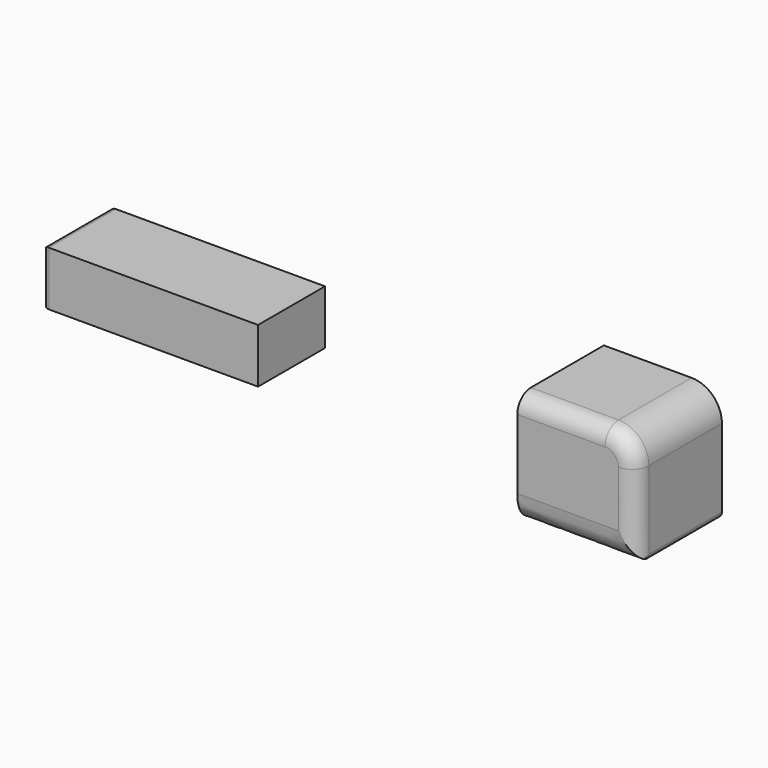
from build123d import *

# Parameters (mm, degrees)
F0_W        = 90.5269756913
F0_H        = 95.6492051482
F1_DEPTH    = 98.806
F2_R        = 25.4
F3_R        = 14.1038356314
F4_T1_DEPTH = 201.2121108887
F5_T1_DEPTH = 101.5149863872
F6_W        = 180.060595274
F6_H        = 70.0388215482
F7_DEPTH    = 45.466
F8_R        = 5.08


# Not quite as in the source:
# - a fillet or chamfer that OpenCascade refuses, or shapes differently, is made with other operations: its cross-section is extruded or revolved along the edge and cut away or added


with BuildPart() as f1:
    # F0 (on Right) → F1 (new body)
    with BuildSketch(Plane.YZ):
        with Locations((0.7718615234, 14.4452676177)):
            Rectangle(F0_W, F0_H)
    extrude(amount=F1_DEPTH)

    # F2
    f2_edges = [f1.edges().sort_by_distance(p)[0] for p in [
        (98.806, 0.771862, 62.26987),
    ]]
    fillet(f2_edges, radius=F2_R)

    # F3
    f3_edges = [f1.edges().sort_by_distance(p)[0] for p in [
        (36.703, -44.491626, 62.26987),
        (91.366512, -44.491626, 54.830382),
        (98.806, -44.491626, 1.745268),
    ]]
    fillet(f3_edges, radius=F3_R)

    # F4: fillet of radius 23.301989304 on 1 edges, made by hand

    # F4_s2 → F4_t1 (cut)
    with BuildSketch(Plane.YZ.offset(-58.2549732601)):
        with BuildLine():
            add(Edge.make_bspline(
                [(-44.4916263223, -10.0773456524), (-44.4916263223, -33.3793349564), (-21.1896370182, -33.3793349564)],
                knots=[0, 0, 0, 1, 1, 1], degree=2, weights=[1, 1, 1]))
            Line((-21.1896370182, -33.3793349564), (-44.4916263223, -33.3793349564))
            Line((-44.4916263223, -33.3793349564), (-44.4916263223, -10.0773456524))
        make_face()
    extrude(amount=F4_T1_DEPTH, mode=Mode.SUBTRACT)

    # F5: fillet of radius 5.08 on 1 edges, made by hand

    # F5_s2 → F5_t1 (cut)
    with BuildSketch(Plane.XZ.offset(-58.735349369)):
        with BuildLine():
            ThreePointArc((98.806, -28.2993349564), (97.3181024484, -31.8914374048), (93.726, -33.3793349564))
            Line((93.726, -33.3793349564), (98.806, -33.3793349564))
            Line((98.806, -33.3793349564), (98.806, -28.2993349564))
        make_face()
    extrude(amount=F5_T1_DEPTH, mode=Mode.SUBTRACT)


with BuildPart() as f7:
    # F6 (on Top) → F7 (new body)
    with BuildSketch(Plane.XY):
        with Locations((-359.2647463083, 55.8701176196)):
            Rectangle(F6_W, F6_H)
    extrude(amount=-F7_DEPTH)

    # F8
    f8_edges = [f7.edges().sort_by_distance(p)[0] for p in [
        (-449.295044, 55.870118, 0),
        (-449.295044, 20.850707, -22.733),
    ]]
    fillet(f8_edges, radius=F8_R)


solid = Compound([f1.part, f7.part])
